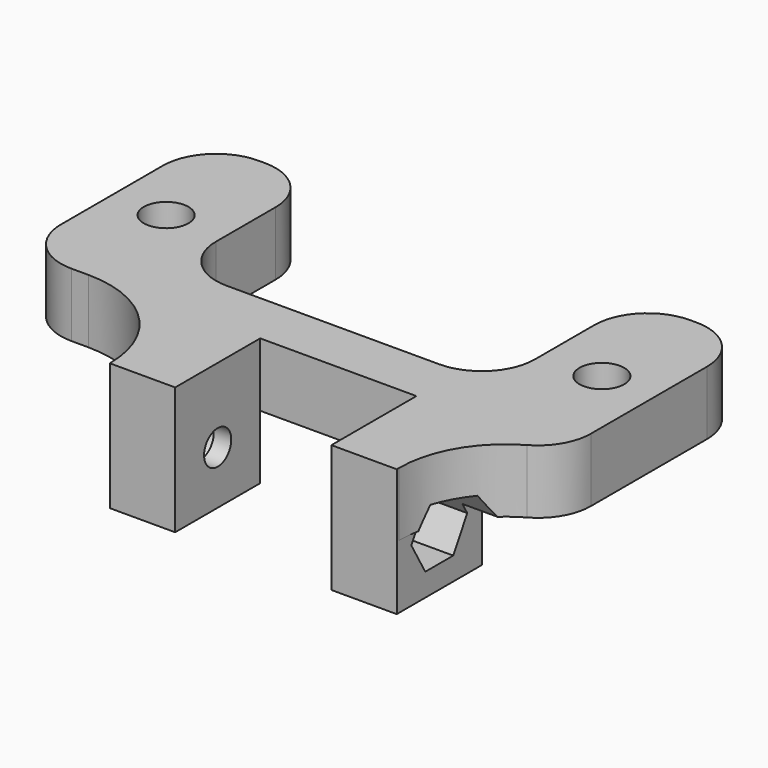
from build123d import *

# Parameters (mm, degrees)
F0_W           = 51.2
F0_H           = 22
F1_DEPTH       = 6
F2_R           = 2.1
F3_DEPTH       = 6.001
F5_DEPTH       = 6.001
F8_DEPTH       = 13.5
F9_W           = 14.7
F9_H           = 10
F10_DEPTH      = 12.001
F11_T1_DEPTH   = 6
F12_R          = 1.6
F13_DEPTH      = 34.601
F13_DEPTH_BACK = 16.601
F14_R          = 2.75
F15_DEPTH      = 4.5
F15_DEPTH_BACK = 16.601
F17_DEPTH      = 4.5
F17_DEPTH_BACK = 25
F18_W          = 30
F18_H          = 17
F19_DEPTH      = 12.001
F20_T1_DEPTH   = 6
F20_T3_DEPTH   = 31
F20_T5_DEPTH   = 22.6993813232


# Not quite as in the source:
# - a fillet or chamfer that OpenCascade refuses, or shapes differently, is made with other operations: its cross-section is extruded or revolved along the edge and cut away or added


with BuildPart() as f1:
    # F0 (on Top) → F1 (new body)
    with BuildSketch(Plane.XY):
        Rectangle(F0_W, F0_H)
    extrude(amount=F1_DEPTH)

    # F2 (on face) → F3 (cut, through all)
    with BuildSketch(Plane.XY.offset(6)):
        with Locations((-20.5, 0)):
            Circle(F2_R)
        with Locations((20.5, 0)):
            Circle(F2_R)
    extrude(amount=-F3_DEPTH, mode=Mode.SUBTRACT)

    # F4 (on face) → F5 (cut, through all)
    with BuildSketch(Plane.XY.offset(6)):
        with BuildLine():
            Line((-1.5, 11), (-1.5, 0))
            ThreePointArc((-1.5, 0), (4.5, -6), (10.5, 0))
            Line((10.5, 0), (10.5, 11))
            Line((10.5, 11), (-1.5, 11))
        make_face()
    extrude(amount=-F5_DEPTH, mode=Mode.SUBTRACT)

    # F7 (on mid) → F8 (join, symmetric)
    with BuildSketch(Plane(origin=(4.5, 0, 0), x_dir=(0, -1, 0), z_dir=(-1, 0, 0))):
        Polygon((21, 6), (11, 6), (11, 0), (11, -6), (21, -6), align=None)
    extrude(amount=F8_DEPTH, both=True)

    # F9 (on face) → F10 (cut, through all)
    with BuildSketch(Plane(origin=(0, 0, -6), x_dir=(1, 0, 0), z_dir=(0, 0, -1))):
        with Locations((4.5, 16)):
            Rectangle(F9_W, F9_H)
    extrude(amount=-F10_DEPTH, mode=Mode.SUBTRACT)

    # F11: fillet of radius 10 on 2 edges, made by hand

    # F11_s2 → F11_t1 (join)
    with BuildSketch(Plane.XY):
        with BuildLine():
            ThreePointArc((-19, -11), (-11.9289321881, -13.9289321881), (-9, -21))
            Line((-9, -21), (-9, -11))
            Line((-9, -11), (-19, -11))
        make_face()
        with BuildLine():
            ThreePointArc((25.6, -11), (20.125992126, -14.5433148766), (18, -20.7077288796))
            Line((18, -20.7077288796), (18, -11))
            Line((18, -11), (25.6, -11))
        make_face()
    extrude(amount=F11_T1_DEPTH)

    # F12 (on face) → F13 (cut, two sides)
    with BuildSketch(Plane(origin=(-9, 0, 0), x_dir=(0, -1, 0), z_dir=(-1, 0, 0))) as f13_sk:
        with Locations((16, -1)):
            Circle(F12_R)
    extrude(amount=-F13_DEPTH, mode=Mode.SUBTRACT)
    extrude(f13_sk.sketch, amount=F13_DEPTH_BACK, mode=Mode.SUBTRACT)

    # F14 (on face) → F15 (cut, two sides)
    with BuildSketch(Plane(origin=(-9, 0, 0), x_dir=(0, -1, 0), z_dir=(-1, 0, 0))) as f15_sk:
        with Locations((16, -1)):
            Circle(F14_R)
    extrude(amount=-F15_DEPTH, mode=Mode.SUBTRACT)
    extrude(f15_sk.sketch, amount=F15_DEPTH_BACK, mode=Mode.SUBTRACT)

    # F16 (on face) → F17 (cut, two sides)
    with BuildSketch(Plane.YZ.offset(18)) as f17_sk:
        Polygon((-14.3545517328, -3.85), (-12.7091034656, -1), (-14.3545517328, 1.85), (-17.6454482672, 1.85), (-19.2908965344, -1), (-17.6454482672, -3.85), align=None)
    extrude(amount=-F17_DEPTH, mode=Mode.SUBTRACT)
    extrude(f17_sk.sketch, amount=F17_DEPTH_BACK, mode=Mode.SUBTRACT)

    # F18 (on face) → F19 (cut, through all)
    with BuildSketch(Plane.XY.offset(6)):
        with Locations((0, 2.5)):
            Rectangle(F18_W, F18_H)
    extrude(amount=-F19_DEPTH, mode=Mode.SUBTRACT)

    # F20: fillet of radius 5 on 9 edges, made by hand

    # F20_s2 → F20_t1 (join)
    with BuildSketch(Plane.XY):
        with BuildLine():
            ThreePointArc((-15, -1), (-13.5355339059, -4.5355339059), (-10, -6))
            Line((-10, -6), (-15, -6))
            Line((-15, -6), (-15, -1))
        make_face()
        with BuildLine():
            ThreePointArc((10, -6), (13.5355339059, -4.5355339059), (15, -1))
            Line((15, -1), (15, -6))
            Line((15, -6), (10, -6))
        make_face()
    extrude(amount=F20_T1_DEPTH)

    # F20_s4 → F20_t3 (cut)
    with BuildSketch(Plane.XY.offset(-12.5)):
        with BuildLine():
            ThreePointArc((-25.6, -6), (-24.1355339059, -9.5355339059), (-20.6, -11))
            Line((-20.6, -11), (-25.6, -11))
            Line((-25.6, -11), (-25.6, -6))
        make_face()
        with BuildLine():
            ThreePointArc((25.6, 6), (24.1355339059, 9.5355339059), (20.6, 11))
            Line((20.6, 11), (25.6, 11))
            Line((25.6, 11), (25.6, 6))
        make_face()
        with BuildLine():
            ThreePointArc((20, 11), (16.4644660941, 9.5355339059), (15, 6))
            Line((15, 6), (15, 11))
            Line((15, 11), (20, 11))
        make_face()
        with BuildLine():
            ThreePointArc((-20.6, 11), (-24.1355339059, 9.5355339059), (-25.6, 6))
            Line((-25.6, 6), (-25.6, 11))
            Line((-25.6, 11), (-20.6, 11))
        make_face()
        with BuildLine():
            ThreePointArc((-15, 6), (-16.4644660941, 9.5355339059), (-20, 11))
            Line((-20, 11), (-15, 11))
            Line((-15, 11), (-15, 6))
        make_face()
    extrude(amount=F20_T3_DEPTH, mode=Mode.SUBTRACT)

    # F20_s6 → F20_t5 (cut)
    with BuildSketch(Plane.XY.offset(-8.3496906616)):
        with BuildLine():
            ThreePointArc((25.6, -7.6601237354), (24.9204937989, -10.1767352138), (23.0666666667, -12.0093254501))
            ThreePointArc((23.0666666667, -12.0093254501), (24.298766569, -11.4179026654), (25.6, -11))
            Line((25.6, -11), (25.6, -7.6601237354))
        make_face()
    extrude(amount=F20_T5_DEPTH, mode=Mode.SUBTRACT)


solid = f1.part
